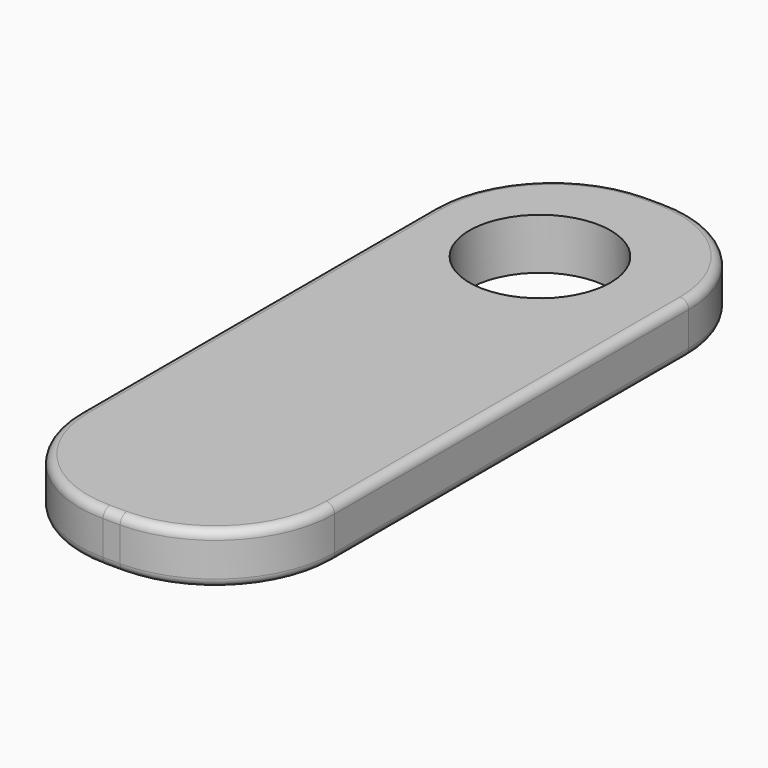
from build123d import *

# Parameters (mm, degrees)
F0_W         = 15
F0_H         = 40
F1_DEPTH     = 3
F2_R         = 0.5
F3_T1_DEPTH  = 3
F3_T4_ANGLE  = 90
F3_T6_ANGLE  = 90
F3_T8_ANGLE  = 90
F3_T10_ANGLE = 90
F3_T12_ANGLE = 90
F3_T14_ANGLE = 90
F3_T16_ANGLE = 90
F3_T18_ANGLE = 90
F4_R         = 4.1479676184
F5_DEPTH     = 25


# Not quite as in the source:
# - a fillet or chamfer that OpenCascade refuses, or shapes differently, is made with other operations: its cross-section is extruded or revolved along the edge and cut away or added


with BuildPart() as f1:
    # F0 (on Top) → F1 (new body)
    with BuildSketch(Plane.XY):
        with Locations((7.5, -20)):
            Rectangle(F0_W, F0_H)
    extrude(amount=F1_DEPTH)

    # F2
    f2_edges = [f1.edges().sort_by_distance(p)[0] for p in [
        (15, -20, 3),
        (7.5, 0, 3),
        (0, -20, 3),
        (7.5, -40, 3),
        (15, -20, 0),
        (7.5, 0, 0),
        (0, -20, 0),
        (7.5, -40, 0),
    ]]
    fillet(f2_edges, radius=F2_R)

    # F3: fillet of radius 7 on 4 edges, made by hand

    # F3_s2 → F3_t1 (cut)
    with BuildSketch(Plane.XY):
        with BuildLine():
            ThreePointArc((15, -7), (12.9497474683, -2.0502525317), (8, 0))
            Line((8, 0), (15, 0))
            Line((15, 0), (15, -7))
        make_face()
        with BuildLine():
            ThreePointArc((7, 0), (2.0502525317, -2.0502525317), (0, -7))
            Line((0, -7), (0, 0))
            Line((0, 0), (7, 0))
        make_face()
        with BuildLine():
            ThreePointArc((15, -33), (12.9497474683, -37.9497474683), (8, -40))
            Line((8, -40), (15, -40))
            Line((15, -40), (15, -33))
        make_face()
        with BuildLine():
            ThreePointArc((7, -40), (2.0502525317, -37.9497474683), (0, -33))
            Line((0, -33), (0, -40))
            Line((0, -40), (7, -40))
        make_face()
    extrude(amount=F3_T1_DEPTH, mode=Mode.SUBTRACT)

    # F3_s3 → F3_t4 (revolve, cut)
    with BuildSketch(Plane.YZ.offset(7)):
        with BuildLine():
            ThreePointArc((-39.5, 0), (-39.8535533906, 0.1464466094), (-40, 0.5))
            Line((-40, 0.5), (-40, 0))
            Line((-40, 0), (-39.5, 0))
        make_face()
    revolve(axis=Axis((7, -33, 0), (0, 0, -1)), revolution_arc=F3_T4_ANGLE, mode=Mode.SUBTRACT)

    # F3_s5 → F3_t6 (revolve, cut)
    with BuildSketch(Plane.XZ.offset(33)):
        with BuildLine():
            ThreePointArc((0.5, 3), (0.1464466094, 2.8535533906), (0, 2.5))
            Line((0, 2.5), (0, 3))
            Line((0, 3), (0.5, 3))
        make_face()
    revolve(axis=Axis((7, -33, 3), (0, 0, 1)), revolution_arc=F3_T6_ANGLE, mode=Mode.SUBTRACT)

    # F3_s7 → F3_t8 (revolve, cut)
    with BuildSketch(Plane.XZ.offset(33)):
        with BuildLine():
            ThreePointArc((14.5, 0), (14.8535533906, 0.1464466094), (15, 0.5))
            Line((15, 0.5), (15, 0))
            Line((15, 0), (14.5, 0))
        make_face()
    revolve(axis=Axis((8, -33, 0), (0, 0, -1)), revolution_arc=F3_T8_ANGLE, mode=Mode.SUBTRACT)

    # F3_s9 → F3_t10 (revolve, cut)
    with BuildSketch(Plane.YZ.offset(8)):
        with BuildLine():
            ThreePointArc((-39.5, 3), (-39.8535533906, 2.8535533906), (-40, 2.5))
            Line((-40, 2.5), (-40, 3))
            Line((-40, 3), (-39.5, 3))
        make_face()
    revolve(axis=Axis((8, -33, 3), (0, 0, 1)), revolution_arc=F3_T10_ANGLE, mode=Mode.SUBTRACT)

    # F3_s11 → F3_t12 (revolve, cut)
    with BuildSketch(Plane.XZ.offset(7)):
        with BuildLine():
            ThreePointArc((0.5, 0), (0.1464466094, 0.1464466094), (0, 0.5))
            Line((0, 0.5), (0, 0))
            Line((0, 0), (0.5, 0))
        make_face()
    revolve(axis=Axis((7, -7, 0), (0, 0, -1)), revolution_arc=F3_T12_ANGLE, mode=Mode.SUBTRACT)

    # F3_s13 → F3_t14 (revolve, cut)
    with BuildSketch(Plane.YZ.offset(7)):
        with BuildLine():
            ThreePointArc((-0.5, 3), (-0.1464466094, 2.8535533906), (0, 2.5))
            Line((0, 2.5), (0, 3))
            Line((0, 3), (-0.5, 3))
        make_face()
    revolve(axis=Axis((7, -7, 3), (0, 0, 1)), revolution_arc=F3_T14_ANGLE, mode=Mode.SUBTRACT)

    # F3_s15 → F3_t16 (revolve, cut)
    with BuildSketch(Plane.YZ.offset(8)):
        with BuildLine():
            ThreePointArc((-0.5, 0), (-0.1464466094, 0.1464466094), (0, 0.5))
            Line((0, 0.5), (0, 0))
            Line((0, 0), (-0.5, 0))
        make_face()
    revolve(axis=Axis((8, -7, 0), (0, 0, -1)), revolution_arc=F3_T16_ANGLE, mode=Mode.SUBTRACT)

    # F3_s17 → F3_t18 (revolve, cut)
    with BuildSketch(Plane.XZ.offset(7)):
        with BuildLine():
            ThreePointArc((14.5, 3), (14.8535533906, 2.8535533906), (15, 2.5))
            Line((15, 2.5), (15, 3))
            Line((15, 3), (14.5, 3))
        make_face()
    revolve(axis=Axis((8, -7, 3), (0, 0, 1)), revolution_arc=F3_T18_ANGLE, mode=Mode.SUBTRACT)

    # F4 (on face) → F5 (cut)
    with BuildSketch(Plane.XY.offset(3)):
        with Locations((6.9764298387, -7.8903073445)):
            Circle(F4_R)
    extrude(amount=-F5_DEPTH, mode=Mode.SUBTRACT)


solid = f1.part
